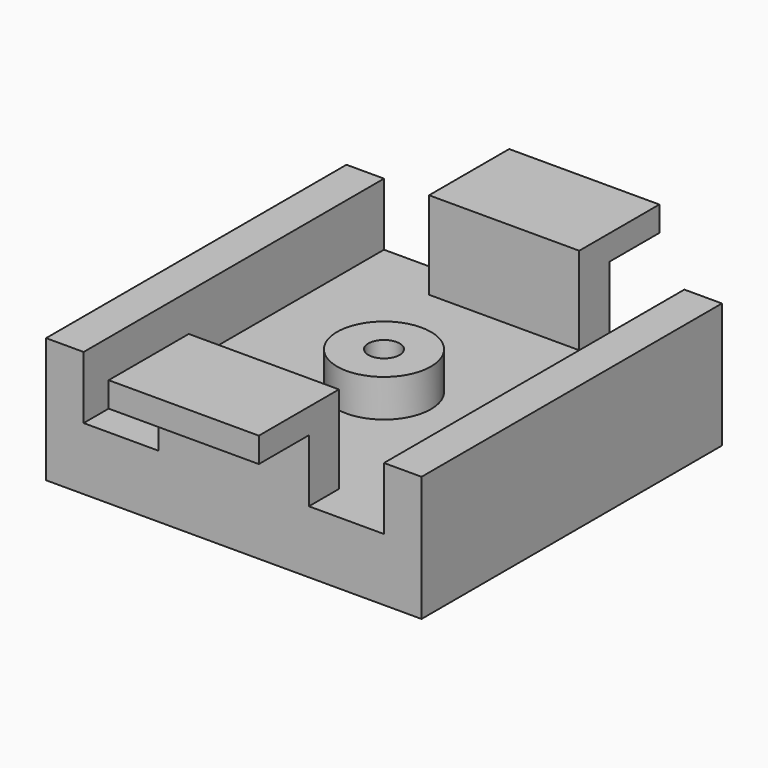
from build123d import *

# Parameters (mm, degrees)
F0_W     = 30
F0_H     = 30
F0_R     = 1.25
F1_DEPTH = 5
F2_W     = 3
F2_H     = 30
F3_DEPTH = 5
F2_R     = 3.75
F2_R_2   = 1.25
F4_DEPTH = 3
F5_W     = 12
F5_H     = 3
F5_H_2   = 5
F6_DEPTH = 2
F7_W     = 12
F7_H     = 5
F7_H_2   = 3
F8_DEPTH = 2


# Not quite as in the source:
# - a feature names something its author has since deleted; it is built from what else it names


with BuildPart() as f1:
    # F0 (on Top) → F1 (new body)
    with BuildSketch(Plane.XY):
        with Locations((15, 15)):
            Rectangle(F0_W, F0_H)
        with Locations((15, 15)):
            Circle(F0_R, mode=Mode.SUBTRACT)
    extrude(amount=F1_DEPTH)

    # F2 (on face) → F3 (join)
    with BuildSketch(Plane.XY.offset(5)):
        with Locations((1.5, 15)):
            Rectangle(F2_W, F2_H)
        with Locations((28.5, 15)):
            Rectangle(F2_W, F2_H)
        Polygon((9, 3), (9, 0), (15, 0), (21, 0), (21, 3), (15, 3), align=None)
        Polygon((15, 30), (9, 30), (9, 27), (15, 27), (21, 27), (21, 30), align=None)
    extrude(amount=F3_DEPTH)

    # F2 (on face) → F4 (join)
    with BuildSketch(Plane.XY.offset(5)):
        with Locations((15, 15)):
            Circle(F2_R)
        with Locations((15, 15)):
            Circle(F2_R_2, mode=Mode.SUBTRACT)
    extrude(amount=F4_DEPTH)

    # F5 (on face) → F6 (join)
    with BuildSketch(Plane.XY.offset(10)):
        with Locations((15, 1.5)):
            Rectangle(F5_W, F5_H)
        with Locations((15, -2.5)):
            Rectangle(F5_W, F5_H_2)
    extrude(amount=F6_DEPTH)

    # F7 (on face) → F8 (join)
    with BuildSketch(Plane.XY.offset(10)):
        with Locations((15, 32.5)):
            Rectangle(F7_W, F7_H)
        with Locations((15, 28.5)):
            Rectangle(F7_W, F7_H_2)
    extrude(amount=F8_DEPTH)


solid = f1.part
